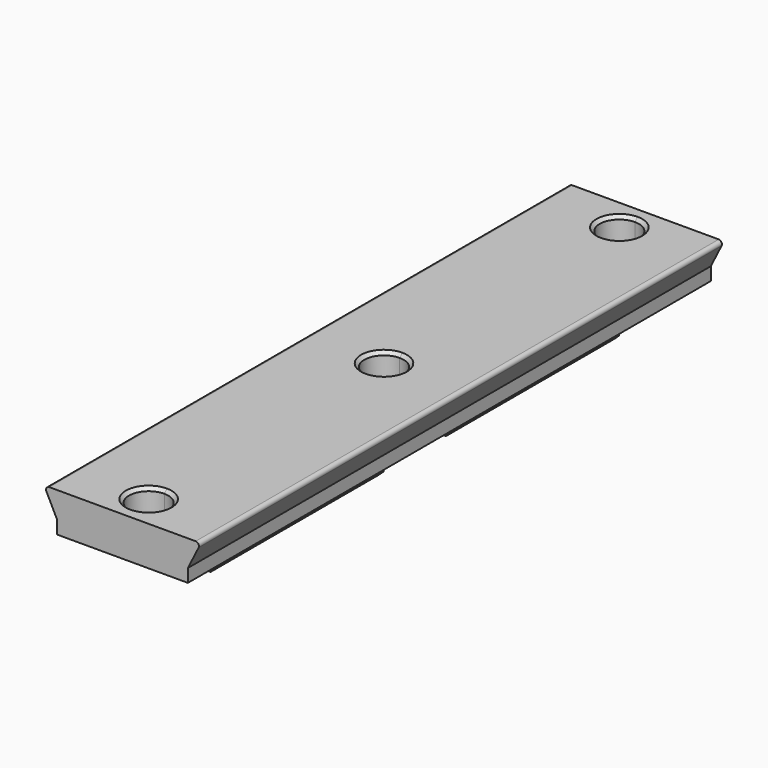
from build123d import *

# Parameters (mm, degrees)
F1_DEPTH  = 100
F2_W      = 5
F2_H      = 10
F3_DEPTH  = 5
F4_R      = 0.9
F5_DEPTH  = 25
F7_DEPTH  = 3.5
F8_DEPTH  = 11.001
F9_SIZE   = 0.5
F10_W     = 11
F10_H     = 5
F10_W_2   = 12
F11_DEPTH = 25
F12_W     = 5
F12_H     = 33
F13_DEPTH = 8
F14_W     = 5
F14_H     = 33
F15_DEPTH = 8
F16_SIZE  = 0.4
F17_R     = 0.5


with BuildPart() as f1:
    # F0 (on Front) → F1 (new body)
    with BuildSketch(Plane.XZ):
        Polygon((2.5, -2.5), (4.75, -2.5), (4.75, 2.5), (10, 2.5), (10, 4.5), (12, 8.5), (10, 8.5), (6, 8.5), (-6, 8.5), (-10, 8.5), (-12, 8.5), (-10, 4.5), (-10, 2.5), (-4.75, 2.5), (-4.75, -2.5), (-2.5, -2.5), (-2.5, 2.5), (2.5, 2.5), align=None)
    extrude(amount=F1_DEPTH)

    # F2 (on face) → F3 (join)
    with BuildSketch(Plane(origin=(0, 0, 2.5), x_dir=(1, 0, 0), z_dir=(0, 0, -1))):
        with Locations((0, 95)):
            Rectangle(F2_W, F2_H)
        Polygon((-2.5, 50), (-2.5, 45), (2.5, 45), (2.5, 50), (2.5, 55), (-2.5, 55), align=None)
        with Locations((0, 5)):
            Rectangle(F2_W, F2_H)
    extrude(amount=F3_DEPTH)

    # F4 (on face) → F5 (cut)
    with BuildSketch(Plane.YZ.offset(4.75)):
        with Locations((-85, 0)):
            Circle(F4_R)
        with Locations((-40, 0)):
            Circle(F4_R)
        with BuildLine():
            ThreePointArc((-14.1, 0), (-15, 0.9), (-15.9, 0))
            Line((-15.9, 0), (-14.1, 0))
        make_face()
        with BuildLine():
            Line((-14.1, 0), (-15.9, 0))
            ThreePointArc((-15.9, 0), (-15, -0.9), (-14.1, 0))
        make_face()
        with Locations((-60, 0)):
            Circle(F4_R)
    extrude(amount=-F5_DEPTH, mode=Mode.SUBTRACT)

    # F6 (on face) → F7 (cut)
    with BuildSketch(Plane.XY.offset(8.5)):
        with BuildLine():
            ThreePointArc((0, -92), (-3, -95), (0, -98))
            Line((0, -98), (0, -96.75))
            ThreePointArc((0, -96.75), (-1.75, -95), (0, -93.25))
            Line((0, -93.25), (0, -92))
        make_face()
        with BuildLine():
            ThreePointArc((0, -2), (-3, -5), (0, -8))
            Line((0, -8), (0, -6.75))
            ThreePointArc((0, -6.75), (-1.75, -5), (0, -3.25))
            Line((0, -3.25), (0, -2))
        make_face()
        with BuildLine():
            Line((0, -6.75), (0, -8))
            ThreePointArc((0, -8), (2.1213203436, -7.1213203436), (3, -5))
            ThreePointArc((3, -5), (2.1213203436, -2.8786796564), (0, -2))
            Line((0, -2), (0, -3.25))
            ThreePointArc((0, -3.25), (1.2374368671, -3.7625631329), (1.75, -5))
            ThreePointArc((1.75, -5), (1.2374368671, -6.2374368671), (0, -6.75))
        make_face()
        with BuildLine():
            ThreePointArc((0, -47), (-3, -50), (0, -53))
            Line((0, -53), (0, -51.75))
            ThreePointArc((0, -51.75), (-1.75, -50), (0, -48.25))
            Line((0, -48.25), (0, -47))
        make_face()
        with BuildLine():
            Line((0, -51.75), (0, -53))
            ThreePointArc((0, -53), (2.1213203436, -52.1213203436), (3, -50))
            ThreePointArc((3, -50), (2.1213203436, -47.8786796564), (0, -47))
            Line((0, -47), (0, -48.25))
            ThreePointArc((0, -48.25), (1.2374368671, -48.7625631329), (1.75, -50))
            ThreePointArc((1.75, -50), (1.2374368671, -51.2374368671), (0, -51.75))
        make_face()
        with BuildLine():
            Line((0, -96.75), (0, -98))
            ThreePointArc((0, -98), (2.1213203436, -97.1213203436), (3, -95))
            ThreePointArc((3, -95), (2.1213203436, -92.8786796564), (0, -92))
            Line((0, -92), (0, -93.25))
            ThreePointArc((0, -93.25), (1.2374368671, -93.7625631329), (1.75, -95))
            ThreePointArc((1.75, -95), (1.2374368671, -96.2374368671), (0, -96.75))
        make_face()
    extrude(amount=-F7_DEPTH, mode=Mode.SUBTRACT)

    # F8 (cut, through all): faces of the model
    f8_faces = [f1.faces().sort_by_distance(p)[0] for p in [
        (0, -5, 8.5),
        (0, -50, 8.5),
        (0, -95, 8.5),
    ]]
    extrude(f8_faces, amount=-F8_DEPTH, mode=Mode.SUBTRACT)

    # F9
    f9_edges = [f1.edges().sort_by_distance(p)[0] for p in [
        (0, -2, 8.5),
        (0, -47, 8.5),
        (0, -92, 8.5),
        (0, -6.75, 5),
        (0, -51.75, 5),
        (0, -96.75, 5),
        (0, -96.75, -2.5),
        (0, -51.75, -2.5),
        (0, -6.75, -2.5),
    ]]
    chamfer(f9_edges, length=F9_SIZE)

    # F10 (on face) → F11 (cut)
    with BuildSketch(Plane(origin=(-4.75, 0, 0), x_dir=(0, -1, 0), z_dir=(-1, 0, 0))):
        with Locations((5.5, 0)):
            Rectangle(F10_W, F10_H)
        with Locations((50, 0)):
            Rectangle(F10_W_2, F10_H)
        with Locations((94.5, 0)):
            Rectangle(F10_W, F10_H)
    extrude(amount=-F11_DEPTH, mode=Mode.SUBTRACT)

    # F12 (on face) → F13 (cut)
    with BuildSketch(Plane(origin=(0, 0, -2.5), x_dir=(1, 0, 0), z_dir=(0, 0, -1))):
        with Locations((0, 72.5)):
            Rectangle(F12_W, F12_H)
    extrude(amount=-F13_DEPTH, mode=Mode.SUBTRACT)

    # F14 (on face) → F15 (cut)
    with BuildSketch(Plane(origin=(0, 0, -2.5), x_dir=(1, 0, 0), z_dir=(0, 0, -1))):
        with Locations((0, 27.5)):
            Rectangle(F14_W, F14_H)
    extrude(amount=-F15_DEPTH, mode=Mode.SUBTRACT)

    # F16
    f16_edges = [f1.edges().sort_by_distance(p)[0] for p in [
        (-3.625, -11, -2.5),
        (-2.5, -27.5, -2.5),
        (-3.625, -44, -2.5),
        (-4.75, -27.5, -2.5),
        (4.75, -27.5, -2.5),
        (3.625, -44, -2.5),
        (2.5, -27.5, -2.5),
        (3.625, -11, -2.5),
        (4.75, -72.5, -2.5),
        (3.625, -89, -2.5),
        (2.5, -72.5, -2.5),
        (3.625, -56, -2.5),
        (-3.625, -56, -2.5),
        (-2.5, -72.5, -2.5),
        (-3.625, -89, -2.5),
        (-4.75, -72.5, -2.5),
        (0, -44, 5.5),
        (-2.5, -27.5, 5.5),
        (0, -11, 5.5),
        (2.5, -27.5, 5.5),
        (0, -89, 5.5),
        (-2.5, -72.5, 5.5),
        (0, -56, 5.5),
        (2.5, -72.5, 5.5),
    ]]
    chamfer(f16_edges, length=F16_SIZE)

    # F17
    f17_edges = [f1.edges().sort_by_distance(p)[0] for p in [
        (12, -50, 8.5),
        (-12, -50, 8.5),
    ]]
    fillet(f17_edges, radius=F17_R)


solid = f1.part
